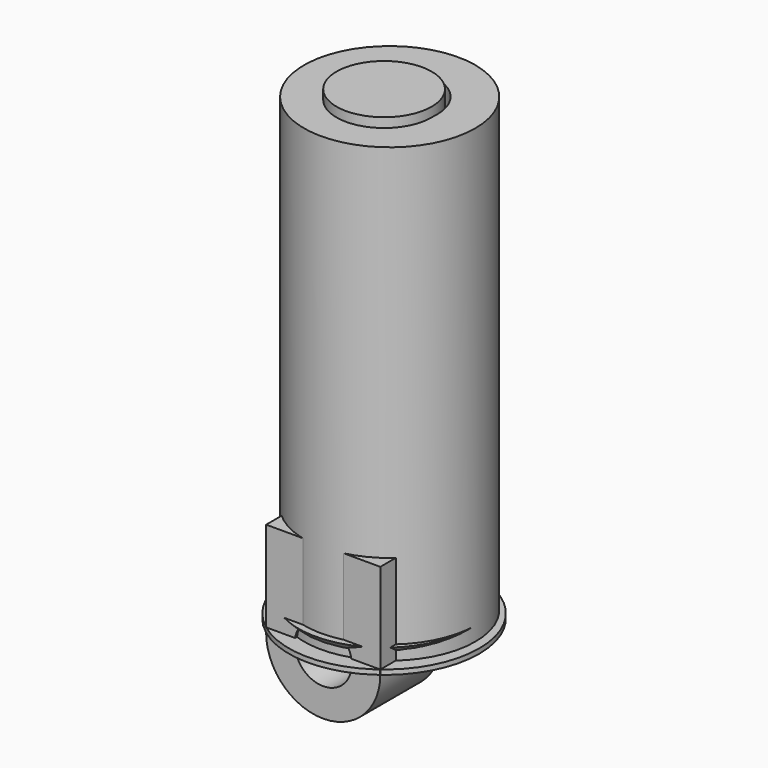
from build123d import *

# Parameters (mm, degrees)
F0_R      = 19.05
F1_DEPTH  = 50.8
F2_R      = 57.15
F3_DEPTH  = 12.7
F4_SIZE   = 12.69999
F5_R      = 63.5
F6_DEPTH  = 3.175
F7_R      = 57.15
F7_R_2    = 31.75
F8_DEPTH  = 304.8
F9_R      = 31.75
F10_DEPTH = 311.15
F12_DEPTH = 12.7


# Not quite as in the source:
# - a fillet or chamfer is up to 0.001 mm smaller than in the source, because OpenCascade refuses the exact size


with BuildPart() as f1:
    # F0 (on Front) → F1 (new body)
    with BuildSketch(Plane.XZ):
        with BuildLine():
            ThreePointArc((-38.1, 0), (0, -38.1), (38.1, 0))
            ThreePointArc((38.1, 0), (0, 38.1), (-38.1, 0))
        make_face()
        Circle(F0_R, mode=Mode.SUBTRACT)
        with BuildLine():
            ThreePointArc((-38.1, 0), (0, 38.1), (38.1, 0))
            Line((38.1, 0), (38.1, 63.5))
            Line((38.1, 63.5), (-38.1, 63.5))
            Line((-38.1, 63.5), (-38.1, 0))
        make_face()
    extrude(amount=F1_DEPTH)


with BuildPart() as f3:
    # F2 (on Top) → F3 (new body)
    with BuildSketch(Plane.XY):
        Circle(F2_R)
    extrude(amount=F3_DEPTH)

    # F4 (size 12.7 in the source; OpenCascade refuses exactly that, so slightly less here)
    f4_edges = [f3.edges().sort_by_distance(p)[0] for p in [
        (-57.15, 0, 0),
    ]]
    chamfer(f4_edges, length=F4_SIZE)


with BuildPart() as f6:
    # F5 (on Top) → F6 (new body)
    with BuildSketch(Plane.XY):
        Circle(F5_R)
    extrude(amount=F6_DEPTH)


with BuildPart() as f8:
    # F7 (on Top) → F8 (new body)
    with BuildSketch(Plane.XY):
        with Locations((0, 4.6629247808)):
            Circle(F7_R)
        with Locations((0, 4.6629247808)):
            Circle(F7_R_2, mode=Mode.SUBTRACT)
    extrude(amount=F8_DEPTH)


with BuildPart() as f10:
    # F9 (on Top) → F10 (new body)
    with BuildSketch(Plane.XY):
        Circle(F9_R)
    extrude(amount=F10_DEPTH)


with BuildPart() as f12:
    # F11 (on Front) → F12 (new body)
    with BuildSketch(Plane.XZ):
        with BuildLine():
            Line((171.1853612941, 141.2297336433), (0, 31.75))
            ThreePointArc((0, 31.75), (-30.9973982261, -6.8719577425), (13.4181298103, -28.7752722384))
            Line((13.4181298103, -28.7752722384), (234.95, 0))
            Line((234.95, 0), (171.1853612941, 141.2297336433))
        make_face()
        with BuildLine():
            ThreePointArc((19.05, 0), (-13.4703841816, -13.4703841816), (0, 19.05))
            ThreePointArc((0, 19.05), (13.4703841816, 13.4703841816), (19.05, 0))
        make_face(mode=Mode.SUBTRACT)
    extrude(amount=F12_DEPTH)


solid = Compound([f1.part, f3.part, f6.part, f8.part, f10.part])
